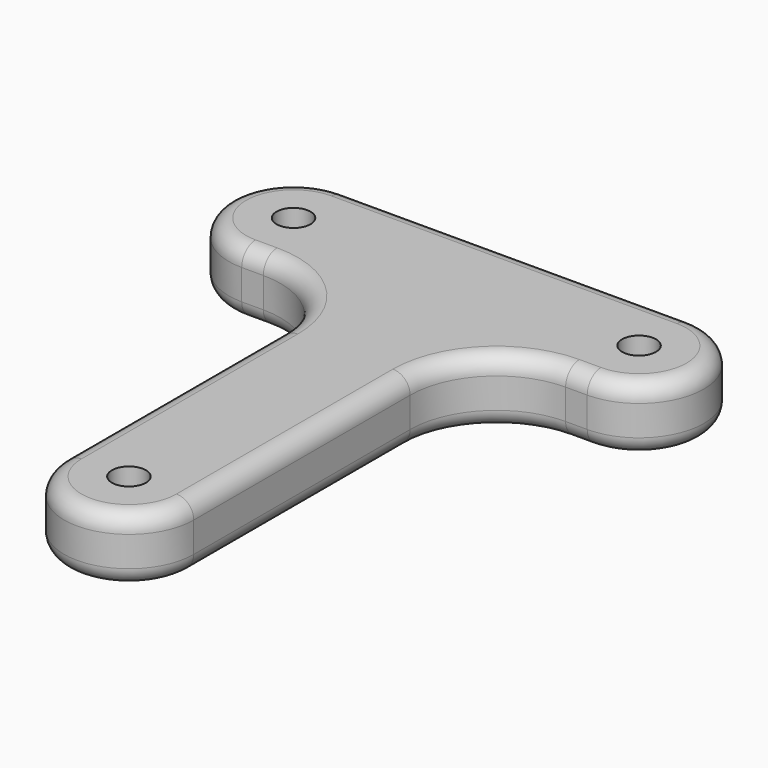
from build123d import *

# Parameters (mm, degrees)
F1_DEPTH = 9.525
F2_D     = 5
F3_R     = 2.54
F4_DEPTH = 4.7


# Not quite as in the source:
# - a feature names something its author has since deleted; it is built from what else it names


with BuildPart() as f1:
    # F0 (on Top) → F1 (new body)
    with BuildSketch(Plane.XY):
        with BuildLine():
            Line((25.4, 29.2563221224), (-25.4, 29.2563221224))
            ThreePointArc((-25.4, 29.2563221224), (-34.925, 19.7313221224), (-25.4, 10.2063221224))
            Line((-25.4, 10.2063221224), (-22.225, 10.2063221224))
            ThreePointArc((-22.225, 10.2063221224), (-13.2447438789, 6.4865782435), (-9.525, -2.4936778776))
            Line((-9.525, -2.4936778776), (-9.525, -42.2686778776))
            ThreePointArc((-9.525, -42.2686778776), (0, -51.7936778776), (9.525, -42.2686778776))
            Line((9.525, -42.2686778776), (9.525, -2.4936778776))
            ThreePointArc((9.525, -2.4936778776), (13.2447438789, 6.4865782435), (22.225, 10.2063221224))
            Line((22.225, 10.2063221224), (25.4, 10.2063221224))
            ThreePointArc((25.4, 10.2063221224), (34.925, 19.7313221224), (25.4, 29.2563221224))
        make_face()
        Polygon((-4.9074772881, -42.2686778776), (-2.4537386441, -38.0186778776), (2.4537386441, -38.0186778776), (4.9074772881, -42.2686778776), (2.4537386441, -46.5186778776), (-2.4537386441, -46.5186778776), align=None, mode=Mode.SUBTRACT)
        Polygon((-20.4925227119, 19.7313221224), (-22.9462613559, 15.4813221224), (-27.8537386441, 15.4813221224), (-30.3074772881, 19.7313221224), (-27.8537386441, 23.9813221224), (-22.9462613559, 23.9813221224), align=None, mode=Mode.SUBTRACT)
        Polygon((30.3074772881, 19.7313221224), (27.8537386441, 15.4813221224), (22.9462613559, 15.4813221224), (20.4925227119, 19.7313221224), (22.9462613559, 23.9813221224), (27.8537386441, 23.9813221224), align=None, mode=Mode.SUBTRACT)
        Polygon((2.4537386441, -38.0186778776), (-2.4537386441, -38.0186778776), (-4.9074772881, -42.2686778776), (-2.4537386441, -46.5186778776), (2.4537386441, -46.5186778776), (4.9074772881, -42.2686778776), align=None)
        Polygon((-27.8537386441, 15.4813221224), (-22.9462613559, 15.4813221224), (-20.4925227119, 19.7313221224), (-22.9462613559, 23.9813221224), (-27.8537386441, 23.9813221224), (-30.3074772881, 19.7313221224), align=None)
        Polygon((22.9462613559, 15.4813221224), (27.8537386441, 15.4813221224), (30.3074772881, 19.7313221224), (27.8537386441, 23.9813221224), (22.9462613559, 23.9813221224), (20.4925227119, 19.7313221224), align=None)
    extrude(amount=F1_DEPTH)

    # F2 (through all)
    with Locations(Plane(origin=(0, 0, 0), x_dir=(1, 0, 0), z_dir=(0, 0, -1))):
        with Locations((25.4, -19.7313221224), (-25.4, -19.7313221224), (0, 42.2686778776)):
            Hole(F2_D / 2)

    # F3
    f3_edges = [f1.edges().sort_by_distance(p)[0] for p in [
        (0, 29.256322, 0),
        (0, 29.256322, 9.525),
    ]]
    fillet(f3_edges, radius=F3_R)

    # F0 (on Top) → F4 (cut)
    with BuildSketch(Plane.XY):
        Polygon((2.4537386441, -38.0186778776), (-2.4537386441, -38.0186778776), (-4.9074772881, -42.2686778776), (-2.4537386441, -46.5186778776), (2.4537386441, -46.5186778776), (4.9074772881, -42.2686778776), align=None)
        Polygon((-27.8537386441, 15.4813221224), (-22.9462613559, 15.4813221224), (-20.4925227119, 19.7313221224), (-22.9462613559, 23.9813221224), (-27.8537386441, 23.9813221224), (-30.3074772881, 19.7313221224), align=None)
        Polygon((22.9462613559, 15.4813221224), (27.8537386441, 15.4813221224), (30.3074772881, 19.7313221224), (27.8537386441, 23.9813221224), (22.9462613559, 23.9813221224), (20.4925227119, 19.7313221224), align=None)
    extrude(amount=F4_DEPTH, mode=Mode.SUBTRACT)


solid = f1.part
